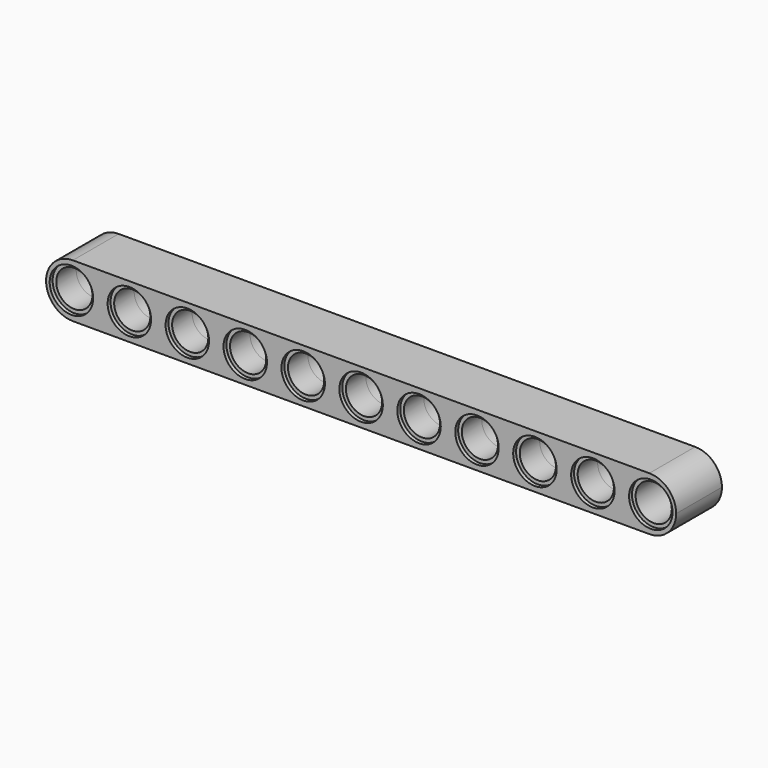
from build123d import *

# Parameters (mm, degrees)
F0_W     = 87
F0_H     = 7.4
F0_R     = 3
F1_DEPTH = 3.95
F0_R_2   = 2.499
F2_DEPTH = 3.45
F3_R     = 3.69999


# Not quite as in the source:
# - a fillet or chamfer is up to 0.001 mm smaller than in the source, because OpenCascade refuses the exact size


with BuildPart() as f1:
    # F0 (on Front) → F1 (new body, symmetric)
    with BuildSketch(Plane.XZ):
        Rectangle(F0_W, F0_H)
        with Locations((-40, 0)):
            Circle(F0_R, mode=Mode.SUBTRACT)
        with Locations((-32, 0)):
            Circle(F0_R, mode=Mode.SUBTRACT)
        with Locations((-24, 0)):
            Circle(F0_R, mode=Mode.SUBTRACT)
        with Locations((-16, 0)):
            Circle(F0_R, mode=Mode.SUBTRACT)
        with Locations((-8, 0)):
            Circle(F0_R, mode=Mode.SUBTRACT)
        Circle(F0_R, mode=Mode.SUBTRACT)
        with Locations((8, 0)):
            Circle(F0_R, mode=Mode.SUBTRACT)
        with Locations((16, 0)):
            Circle(F0_R, mode=Mode.SUBTRACT)
        with Locations((24, 0)):
            Circle(F0_R, mode=Mode.SUBTRACT)
        with Locations((32, 0)):
            Circle(F0_R, mode=Mode.SUBTRACT)
        with Locations((40, 0)):
            Circle(F0_R, mode=Mode.SUBTRACT)
    extrude(amount=F1_DEPTH, both=True)

    # F0 (on Front) → F2 (join, symmetric)
    with BuildSketch(Plane.XZ):
        with Locations((-40, 0)):
            Circle(F0_R)
        with Locations((-40, 0)):
            Circle(F0_R_2, mode=Mode.SUBTRACT)
        with Locations((-32, 0)):
            Circle(F0_R)
        with Locations((-32, 0)):
            Circle(F0_R_2, mode=Mode.SUBTRACT)
        with Locations((-24, 0)):
            Circle(F0_R)
        with Locations((-24, 0)):
            Circle(F0_R_2, mode=Mode.SUBTRACT)
        with Locations((-16, 0)):
            Circle(F0_R)
        with Locations((-16, 0)):
            Circle(F0_R_2, mode=Mode.SUBTRACT)
        with Locations((-8, 0)):
            Circle(F0_R)
        with Locations((-8, 0)):
            Circle(F0_R_2, mode=Mode.SUBTRACT)
        Circle(F0_R)
        Circle(F0_R_2, mode=Mode.SUBTRACT)
        with Locations((8, 0)):
            Circle(F0_R)
        with Locations((8, 0)):
            Circle(F0_R_2, mode=Mode.SUBTRACT)
        with Locations((16, 0)):
            Circle(F0_R)
        with Locations((16, 0)):
            Circle(F0_R_2, mode=Mode.SUBTRACT)
        with Locations((24, 0)):
            Circle(F0_R)
        with Locations((24, 0)):
            Circle(F0_R_2, mode=Mode.SUBTRACT)
        with Locations((32, 0)):
            Circle(F0_R)
        with Locations((32, 0)):
            Circle(F0_R_2, mode=Mode.SUBTRACT)
        with Locations((40, 0)):
            Circle(F0_R)
        with Locations((40, 0)):
            Circle(F0_R_2, mode=Mode.SUBTRACT)
    extrude(amount=F2_DEPTH, both=True)

    # F3 (radius 3.7 in the source; OpenCascade refuses exactly that, so slightly less here)
    f3_edges = [f1.edges().sort_by_distance(p)[0] for p in [
        (-43.5, 0, 3.7),
        (-43.5, 0, -3.7),
        (43.5, 0, 3.7),
        (43.5, 0, -3.7),
    ]]
    fillet(f3_edges, radius=F3_R)


solid = f1.part
